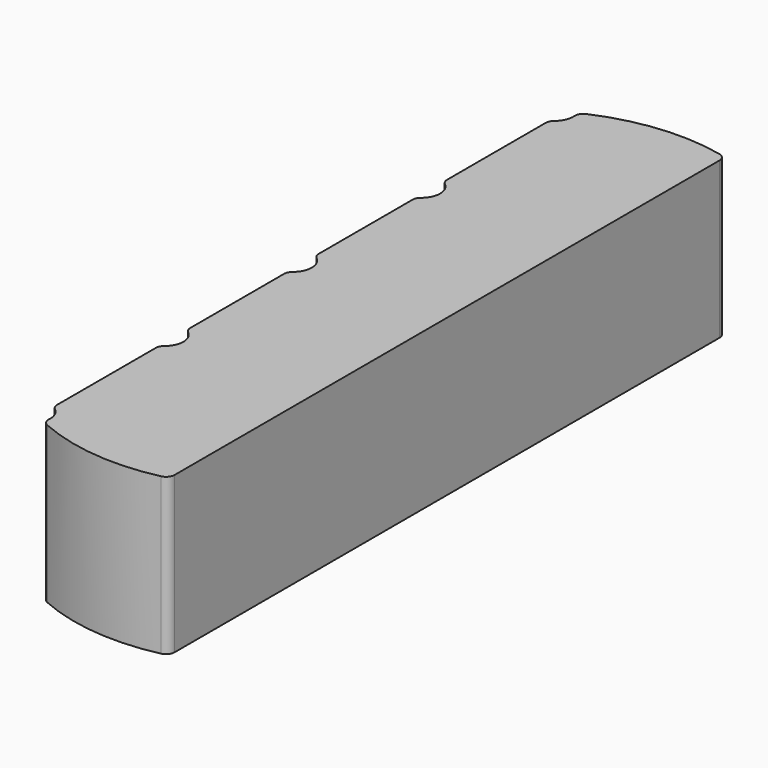
from build123d import *

# Parameters (mm, degrees)
F1_DEPTH = 114.3
F2_T     = -2.032


# Not quite as in the source:
# - ends of sketch curves that miss each other by under 0.0002 mm in the source are joined


with BuildPart() as f1:
    # F0 (on Top) → F1 (new body)
    with BuildSketch(Plane.XY):
        with BuildLine():
            ThreePointArc((-56.5356683944, -224.3892894538), (-55.638228484, -228.1244435583), (-52.7512582129, -230.658645056))
            ThreePointArc((-52.7512582129, -230.658645056), (-8.2827450913, -242.2571362771), (37.5884612507, -239.4631988056))
            ThreePointArc((37.5884612507, -239.4631988056), (41.1635822204, -237.2376139869), (42.5600166876, -233.2646190823))
            Line((42.5600166876, -233.2646190823), (42.5600166876, 15.9969440547))
            Line((42.5600166876, 15.9969440547), (42.5600166876, 16.0075028557))
            Line((42.5600166876, 16.0075028557), (42.5600166876, 265.2690659926))
            ThreePointArc((42.5600166876, 265.2690659926), (41.1635822204, 269.2420608973), (37.5884612507, 271.467645716))
            ThreePointArc((37.5884612507, 271.467645716), (-8.2827450913, 274.2615831875), (-52.7512582129, 262.6630919663))
            ThreePointArc((-52.7512582129, 262.6630919663), (-55.638228484, 260.1288904686), (-56.5356683944, 256.3937363641))
            ThreePointArc((-56.5356683944, 256.3937363641), (-57.6694537634, 249.8005581937), (-61.7387333124, 244.4905269695))
            ThreePointArc((-61.7387333124, 244.4905269695), (-63.4937959622, 242.2831904653), (-64.1199833124, 239.5335598083))
            Line((-64.1199833124, 239.5335598083), (-64.1199833124, 149.3381496402))
            ThreePointArc((-64.1199833124, 149.3381496402), (-63.4937959622, 146.5885189832), (-61.7387333124, 144.3811824789))
            ThreePointArc((-61.7387333124, 144.3811824789), (-56.4999833124, 133.4758547242), (-61.7387333124, 122.5705269695))
            ThreePointArc((-61.7387333124, 122.5705269695), (-63.4937959622, 120.3631904653), (-64.1199833124, 117.6135598083))
            Line((-64.1199833124, 117.6135598083), (-64.1199833124, 31.8632195798))
            ThreePointArc((-64.1199833124, 31.8632195798), (-63.4937959622, 29.1135889227), (-61.7387333124, 26.9062524185))
            ThreePointArc((-61.7387333124, 26.9062524185), (-57.8871404165, 22.0699414424), (-56.5000526478, 16.044938603))
            ThreePointArc((-56.5000526478, 16.044938603), (-56.4999833728, 16.0022234616), (-56.5000526478, 15.9595083074))
            ThreePointArc((-56.5000526478, 15.9595083074), (-57.8871404165, 9.9345054679), (-61.7387333124, 5.0981944918))
            ThreePointArc((-61.7387333124, 5.0981944918), (-63.4937959622, 2.8908579876), (-64.1199833124, 0.1412273306))
            Line((-64.1199833124, 0.1412273306), (-64.1199833124, -85.609112898))
            ThreePointArc((-64.1199833124, -85.609112898), (-63.4937959622, -88.358743555), (-61.7387333124, -90.5660800592))
            ThreePointArc((-61.7387333124, -90.5660800592), (-56.4999833124, -101.4714078139), (-61.7387333124, -112.3767355686))
            ThreePointArc((-61.7387333124, -112.3767355686), (-63.4937959622, -114.5840720728), (-64.1199833124, -117.3337027298))
            Line((-64.1199833124, -117.3337027298), (-64.1199833124, -207.529112898))
            ThreePointArc((-64.1199833124, -207.529112898), (-63.4937959622, -210.278743555), (-61.7387333124, -212.4860800592))
            ThreePointArc((-61.7387333124, -212.4860800592), (-57.6694537634, -217.7961112834), (-56.5356683944, -224.3892894538))
        make_face()
    extrude(amount=F1_DEPTH)

    # F2
    f2_openings = [f1.faces().sort_by_distance(p)[0] for p in [
        (-9.762898, 16.002223, 0),
    ]]
    offset(amount=F2_T, openings=f2_openings, kind=Kind.INTERSECTION)


solid = f1.part
